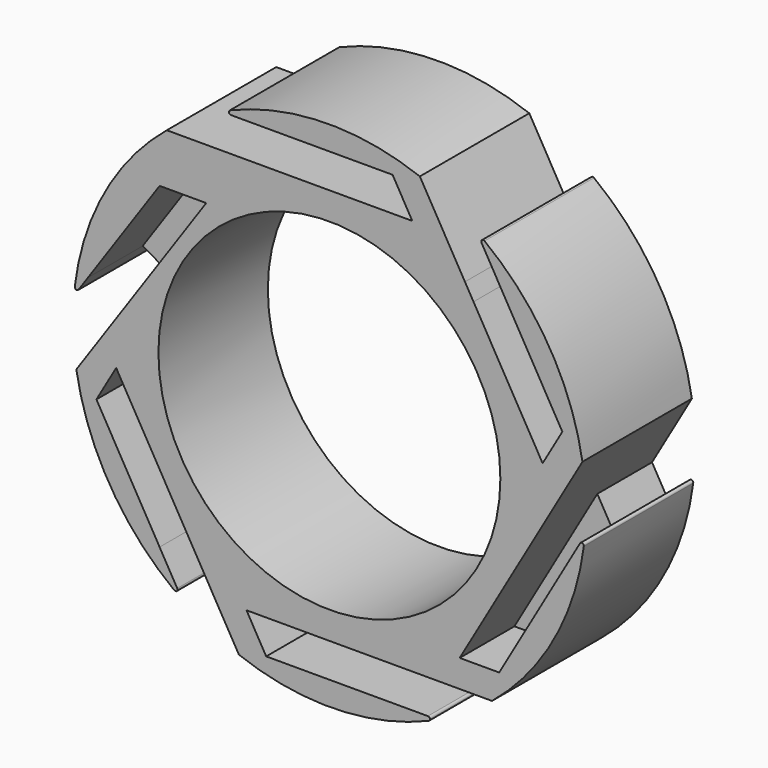
from build123d import *

# Parameters (mm, degrees)
F0_R     = 31.75
F1_DEPTH = 25.4
F2_DEPTH = 12.7
F3_R     = 0.381


# Not quite as in the source:
# - a feature names something its author has since deleted; it is built from what else it names


with BuildPart() as f1:
    # F0 (on Front) → F1 (new body)
    with BuildSketch(Plane.XZ):
        with BuildLine():
            Line((15.3979316793, -36.83), (30.194233307, -36.83))
            ThreePointArc((30.194233307, -36.83), (42.108212504, -22.2494733583), (47.4402273678, -4.1911158763))
            Line((47.4402273678, -4.1911158763), (43.2608556704, -11.43))
            Line((43.2608556704, -11.43), (31.5290982004, -31.75))
            Line((31.5290982004, -31.75), (27.8629239911, -31.75))
            Line((27.8629239911, -31.75), (24.1967497817, -31.75))
            Line((24.1967497817, -31.75), (39.594681461, -5.08))
            Line((39.594681461, -5.08), (46.9928322749, 7.7339730917))
            ThreePointArc((46.9928322749, 7.7339730917), (40.3227154011, 25.3420450573), (27.349726503, 38.9888841237))
            Line((27.349726503, 38.9888841237), (30.6748353416, 33.2296266746))
            Line((30.6748353416, 33.2296266746), (34.095420147, 27.305))
            Line((34.095420147, 27.305), (43.2608556704, 11.43))
            Line((43.2608556704, 11.43), (41.4277685657, 8.255))
            Line((41.4277685657, 8.255), (39.594681461, 5.08))
            Line((39.594681461, 5.08), (26.7630717283, 27.305))
            Line((26.7630717283, 27.305), (25.1755740867, 30.0546265722))
            Line((25.1755740867, 30.0546265722), (16.7985989679, 44.5639730917))
            ThreePointArc((16.7985989679, 44.5639730917), (-1.7854971029, 47.5915184155), (-20.0905008648, 43.18))
            Line((-20.0905008648, 43.18), (-11.7317574699, 43.18))
            Line((-11.7317574699, 43.18), (11.7317574699, 43.18))
            Line((11.7317574699, 43.18), (13.5648445746, 40.005))
            Line((13.5648445746, 40.005), (15.3979316793, 36.83))
            Line((15.3979316793, 36.83), (-15.3979316793, 36.83))
            Line((-15.3979316793, 36.83), (-30.194233307, 36.83))
            ThreePointArc((-30.194233307, 36.83), (-42.108212504, 22.2494733583), (-47.4402273678, 4.1911158763))
            Line((-47.4402273678, 4.1911158763), (-44.833398728, 7.9780209084))
            Line((-44.833398728, 7.9780209084), (-31.5290982004, 27.305))
            Line((-31.5290982004, 27.305), (-27.2009059294, 27.305))
            Line((-27.2009059294, 27.305), (-22.8727136583, 27.305))
            Line((-22.8727136583, 27.305), (-38.6030217944, 4.4537921653))
            Line((-38.6030217944, 4.4537921653), (-46.9928322749, -7.7339730917))
            ThreePointArc((-46.9928322749, -7.7339730917), (-40.3227154011, -25.3420450573), (-27.349726503, -38.9888841237))
            Line((-27.349726503, -38.9888841237), (-31.5290982004, -31.75))
            Line((-31.5290982004, -31.75), (-43.2608556704, -11.43))
            Line((-43.2608556704, -11.43), (-41.4277685657, -8.255))
            Line((-41.4277685657, -8.255), (-39.594681461, -5.08))
            Line((-39.594681461, -5.08), (-24.1967497817, -31.75))
            Line((-24.1967497817, -31.75), (-16.7985989679, -44.5639730917))
            ThreePointArc((-16.7985989679, -44.5639730917), (1.7854971029, -47.5915184155), (20.0905008648, -43.18))
            Line((20.0905008648, -43.18), (11.7317574699, -43.18))
            Line((11.7317574699, -43.18), (-11.7317574699, -43.18))
            Line((-11.7317574699, -43.18), (-13.5648445746, -40.005))
            Line((-13.5648445746, -40.005), (-15.3979316793, -36.83))
            Line((-15.3979316793, -36.83), (15.3979316793, -36.83))
        make_face()
        Circle(F0_R, mode=Mode.SUBTRACT)
    extrude(amount=F1_DEPTH)

    # F0 (on Front) → F2 (join)
    with BuildSketch(Plane.XZ):
        Polygon((-41.7182102612, 6.2159065369), (-38.6030217944, 4.4537921653), (-22.8727136583, 27.305), (-27.2009059294, 27.305), align=None)
        Polygon((-44.833398728, 7.9780209084), (-41.7182102612, 6.2159065369), (-27.2009059294, 27.305), (-31.5290982004, 27.305), align=None)
        Polygon((-27.8629239911, -31.75), (-24.1967497817, -31.75), (-39.594681461, -5.08), (-41.4277685657, -8.255), align=None)
        Polygon((-31.5290982004, -31.75), (-27.8629239911, -31.75), (-41.4277685657, -8.255), (-43.2608556704, -11.43), align=None)
        Polygon((13.5648445746, -40.005), (15.3979316793, -36.83), (-15.3979316793, -36.83), (-13.5648445746, -40.005), align=None)
        Polygon((11.7317574699, -43.18), (13.5648445746, -40.005), (-13.5648445746, -40.005), (-11.7317574699, -43.18), align=None)
        Polygon((27.8629239911, -31.75), (41.4277685657, -8.255), (39.594681461, -5.08), (24.1967497817, -31.75), align=None)
        Polygon((31.5290982004, -31.75), (43.2608556704, -11.43), (41.4277685657, -8.255), (27.8629239911, -31.75), align=None)
        Polygon((43.2608556704, 11.43), (34.095420147, 27.305), (30.4292459376, 27.305), (41.4277685657, 8.255), align=None)
        Polygon((41.4277685657, 8.255), (30.4292459376, 27.305), (26.7630717283, 27.305), (39.594681461, 5.08), align=None)
        Polygon((13.5648445746, 40.005), (-13.5648445746, 40.005), (-15.3979316793, 36.83), (15.3979316793, 36.83), align=None)
        Polygon((11.7317574699, 43.18), (-11.7317574699, 43.18), (-13.5648445746, 40.005), (13.5648445746, 40.005), align=None)
    extrude(amount=F2_DEPTH)

    # F3
    f3_edges = [f1.edges().sort_by_distance(p)[0] for p in [
        (-47.440227, -12.7, 4.191116),
        (-27.349727, -12.7, -38.988884),
        (20.090501, -12.7, -43.18),
        (47.440227, -12.7, -4.191116),
        (27.349727, -12.7, 38.988884),
        (-20.090501, -12.7, 43.18),
    ]]
    fillet(f3_edges, radius=F3_R)


solid = f1.part
